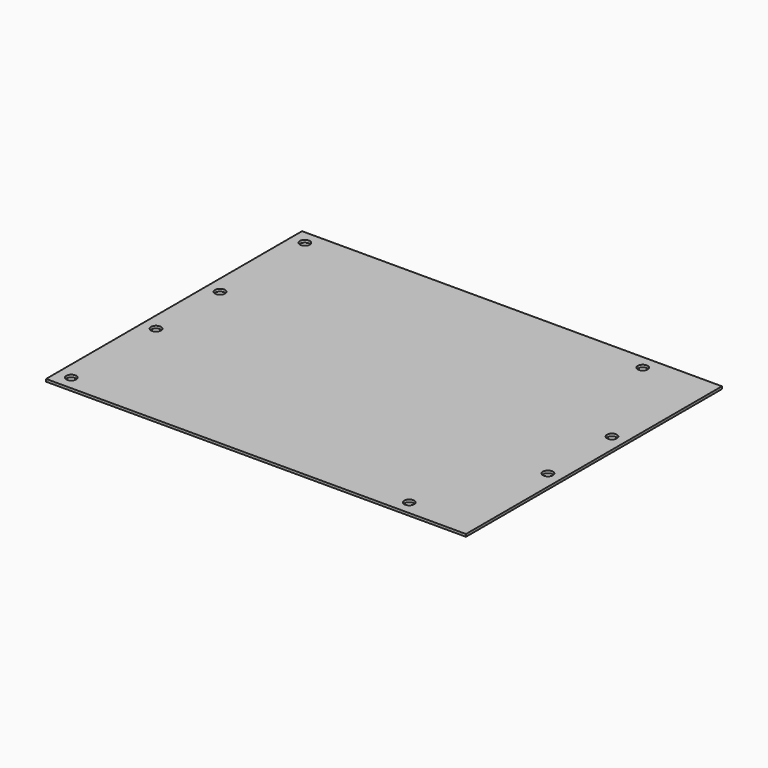
from build123d import *

# Parameters (mm, degrees)
F0_W     = 266.7
F0_H     = 203.2
F0_R     = 3.175
F1_DEPTH = 1.5875


# Not quite as in the source:
# - a length typed as a fraction of an inch, garbled in the dataset ("3 / 203.2 mm" for 3/8 in), is restored


with BuildPart() as f1:
    # F0 (on Top) → F1 (new body)
    with BuildSketch(Plane.XY):
        Rectangle(F0_W, F0_H)
        with Locations((-124.46, -92.71)):
            Circle(F0_R, mode=Mode.SUBTRACT)
        with Locations((-124.46, -25.4)):
            Circle(F0_R, mode=Mode.SUBTRACT)
        with Locations((90.17, -92.71)):
            Circle(F0_R, mode=Mode.SUBTRACT)
        with Locations((124.46, -25.4)):
            Circle(F0_R, mode=Mode.SUBTRACT)
        with Locations((-124.46, 25.4)):
            Circle(F0_R, mode=Mode.SUBTRACT)
        with Locations((-124.46, 92.71)):
            Circle(F0_R, mode=Mode.SUBTRACT)
        with Locations((124.46, 25.4)):
            Circle(F0_R, mode=Mode.SUBTRACT)
        with Locations((90.17, 92.71)):
            Circle(F0_R, mode=Mode.SUBTRACT)
    extrude(amount=F1_DEPTH)


solid = f1.part
